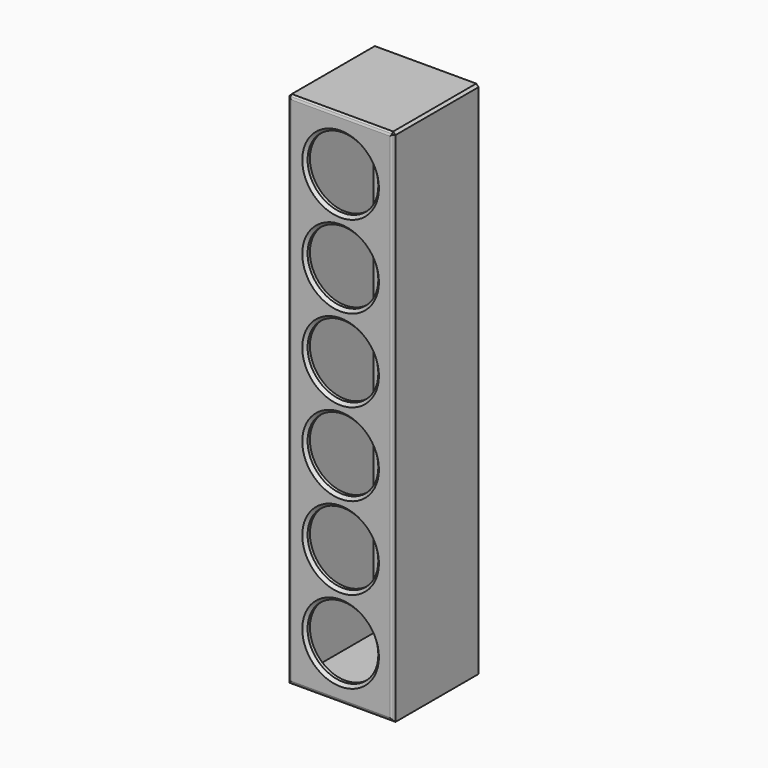
from build123d import *

# Parameters (mm, degrees)
F0_W        = 228.6
F0_H        = 1117.6
F1_DEPTH    = 12.7
F3_DEPTH    = 203.2
F4_W        = 114.3
F4_H        = 1117.6
F5_DEPTH    = 12.7
F7_D        = 152.4
F7_DEPTH    = 25.4
F7_TIP      = 45.7855791699
F8_SIZE     = 5.08
F9_T1_DEPTH = 232.7728499247
F9_T3_DEPTH = 1121.7728499247


# Not quite as in the source:
# - a fillet or chamfer that OpenCascade refuses, or shapes differently, is made with other operations: its cross-section is extruded or revolved along the edge and cut away or added


with BuildPart() as f1:
    # F0 (on Front) → F1 (new body)
    with BuildSketch(Plane.XZ):
        Rectangle(F0_W, F0_H)
    extrude(amount=F1_DEPTH)

    # F2 (on face) → F3 (join)
    with BuildSketch(Plane.XZ.offset(12.7)):
        Polygon((-101.6, 546.1), (-114.3, 558.8), (-114.3, -558.8), (-101.6, -546.1), align=None)
        Polygon((114.3, 558.8), (-114.3, 558.8), (-101.6, 546.1), (101.6, 546.1), align=None)
        Polygon((114.3, -558.8), (114.3, 558.8), (101.6, 546.1), (101.6, -546.1), align=None)
        Polygon((-101.6, -546.1), (-114.3, -558.8), (114.3, -558.8), (101.6, -546.1), align=None)
    extrude(amount=F3_DEPTH)

    # F4 (on face) → F5 (join)
    with BuildSketch(Plane.XZ.offset(215.9)):
        with Locations((-57.15, 0)):
            Rectangle(F4_W, F4_H)
        with Locations((57.15, 0)):
            Rectangle(F4_W, F4_H)
    extrude(amount=F5_DEPTH)

    # F7
    with Locations(Plane.XZ.offset(228.6)):
        with Locations((0, -444.5), (0, -266.7), (0, -88.9), (0, 88.9), (0, 266.7), (0, 444.5)):
            Hole(F7_D / 2, depth=F7_DEPTH)
            with Locations((0, 0, -(F7_DEPTH + F7_TIP / 2))):  # 118° drill point
                Cone(0, F7_D / 2, F7_TIP, mode=Mode.SUBTRACT)

    # F8
    f8_edges = [f1.edges().sort_by_distance(p)[0] for p in [
        (0, -228.6, -558.8),
        (114.3, -228.6, 0),
        (-114.3, -228.6, 0),
        (0, -228.6, 558.8),
        (-114.3, -114.3, 558.8),
        (114.3, -114.3, 558.8),
    ]]
    chamfer(f8_edges, length=F8_SIZE)

    # F9: chamfer of 6.35 on 10 edges, made by hand

    # F9_s2 → F9_t1 (cut)
    with BuildSketch(Plane.YZ.offset(-116.3864249623)):
        Polygon((-226.7401280605, -555.5798719395), (-228.6, -551.0897438789), (-228.6, -553.72), align=None)
        Polygon((-228.6, 551.0897438789), (-226.7401280605, 555.5798719395), (-228.6, 553.72), align=None)
    extrude(amount=F9_T1_DEPTH, mode=Mode.SUBTRACT)

    # F9_s4 → F9_t3 (cut)
    with BuildSketch(Plane.XY.offset(-560.8864249623)):
        Polygon((-106.5897438789, -228.6), (-111.0798719395, -226.7401280605), (-109.22, -228.6), align=None)
        Polygon((111.0798719395, -226.7401280605), (106.5897438789, -228.6), (109.22, -228.6), align=None)
    extrude(amount=F9_T3_DEPTH, mode=Mode.SUBTRACT)

    # F9_s5 → F9_t6 (revolve, cut)
    with BuildSketch(Plane.XY.offset(-444.5)):
        Polygon((82.55, -228.6), (76.2, -222.25), (76.2, -228.6), align=None)
    revolve(axis=Axis((0, -228.6, -444.5), (0, -1, 0)), mode=Mode.SUBTRACT)

    # F9_s7 → F9_t8 (revolve, cut)
    with BuildSketch(Plane.XY.offset(-266.7)):
        Polygon((82.55, -228.6), (76.2, -222.25), (76.2, -228.6), align=None)
    revolve(axis=Axis((0, -228.6, -266.7), (0, -1, 0)), mode=Mode.SUBTRACT)

    # F9_s9 → F9_t10 (revolve, cut)
    with BuildSketch(Plane.XY.offset(-88.9)):
        Polygon((82.55, -228.6), (76.2, -222.25), (76.2, -228.6), align=None)
    revolve(axis=Axis((0, -228.6, -88.9), (0, -1, 0)), mode=Mode.SUBTRACT)

    # F9_s11 → F9_t12 (revolve, cut)
    with BuildSketch(Plane.XY.offset(88.9)):
        Polygon((82.55, -228.6), (76.2, -222.25), (76.2, -228.6), align=None)
    revolve(axis=Axis((0, -228.6, 88.9), (0, -1, 0)), mode=Mode.SUBTRACT)

    # F9_s13 → F9_t14 (revolve, cut)
    with BuildSketch(Plane.XY.offset(266.7)):
        Polygon((82.55, -228.6), (76.2, -222.25), (76.2, -228.6), align=None)
    revolve(axis=Axis((0, -228.6, 266.7), (0, -1, 0)), mode=Mode.SUBTRACT)

    # F9_s15 → F9_t16 (revolve, cut)
    with BuildSketch(Plane.XY.offset(444.5)):
        Polygon((82.55, -228.6), (76.2, -222.25), (76.2, -228.6), align=None)
    revolve(axis=Axis((0, -228.6, 444.5), (0, -1, 0)), mode=Mode.SUBTRACT)


solid = f1.part
